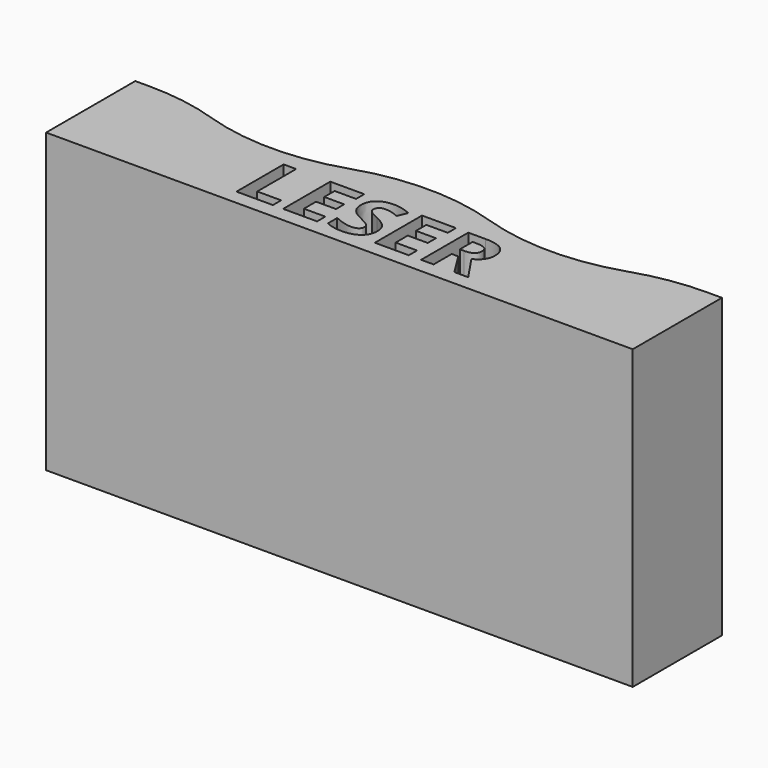
from build123d import *

# Parameters (mm, degrees)
F1_DEPTH     = 40
F2_TEXT_SIZE = 11.1111111111
F3_DEPTH     = 40


# Not quite as in the source:
# - Text() gives the source's letters only with a copy of the font that has no kerning and outlines rounded to 1/6400 em; it was checked with that copy


with BuildPart() as f1:
    # F0 (on Top) → F1 (new body)
    with BuildSketch(Plane.XY):
        with BuildLine():
            Line((0, 15), (0, 0))
            Line((0, 0), (78.936, 0))
            Line((78.936, 0), (78.936, 15))
            Line((78.936, 15), (76.936, 15))
            ThreePointArc((76.936, 15), (72.1928417965, 14.622667845), (67.569, 13.5001633504))
            ThreePointArc((67.569, 13.5001633504), (58.202, 12.0003267008), (48.835, 13.5001633504))
            ThreePointArc((48.835, 13.5001633504), (39.468, 15), (30.101, 13.5001633504))
            ThreePointArc((30.101, 13.5001633504), (20.734, 12.0003267008), (11.367, 13.5001633504))
            ThreePointArc((11.367, 13.5001633504), (6.7431582035, 14.622667845), (2, 15))
            Line((2, 15), (0, 15))
        make_face()
    extrude(amount=F1_DEPTH)

    # F2 (on Top) → F3 (cut)
    with BuildSketch(Plane.XY):
        with Locations((23.019, 2)):
            Text('LESER', F2_TEXT_SIZE, font='Open Sans', font_style=FontStyle.BOLD, text_align=(TextAlign.LEFT, TextAlign.BOTTOM))
    extrude(amount=F3_DEPTH, mode=Mode.SUBTRACT)


solid = f1.part
